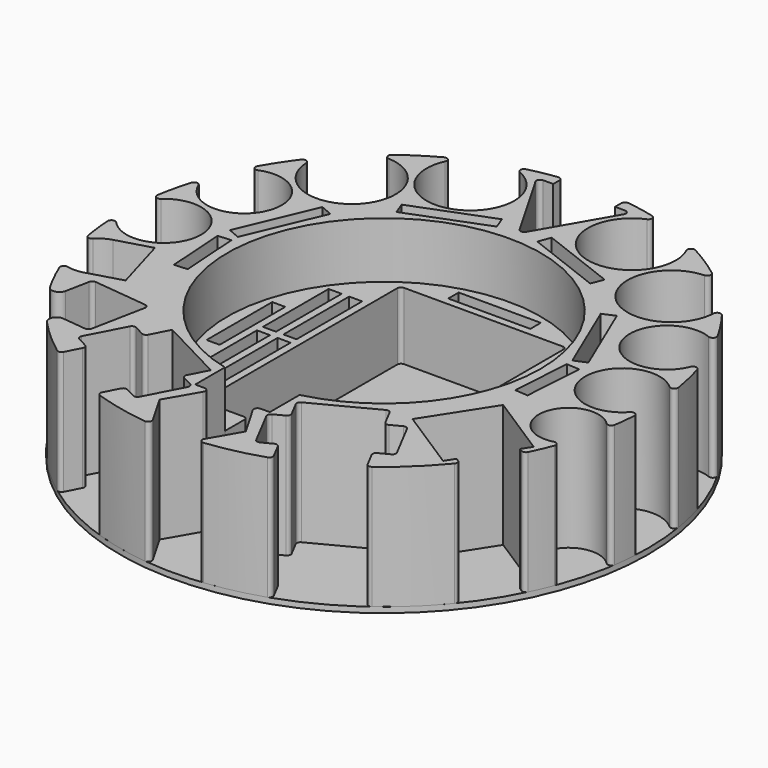
from build123d import *

# Parameters (mm, degrees)
F0_W     = 3.5
F0_H     = 22
F0_W_2   = 22
F0_H_2   = 3.5
F1_DEPTH = 18
F2_R     = 1
F3_DEPTH = 33
F4_R     = 1
F5_DEPTH = 5
F6_R     = 2
F7_R     = 70.7060990639
F8_DEPTH = 1.5


# Not quite as in the source:
# - a feature names something its author has since deleted; it is built from what else it names


with BuildPart() as f1:
    # F0 (on Top) → F1 (new body)
    with BuildSketch(Plane.XY):
        with BuildLine():
            Line((-22.25, -33.25), (-22.25, 33.25))
            Line((-22.25, 33.25), (22.25, 33.25))
            Line((22.25, 33.25), (22.25, -33.25))
            Line((22.25, -33.25), (10, -33.25))
            Line((10, -33.25), (10, -40.7921561087))
            ThreePointArc((10, -40.7921561087), (33.0454232837, -25.9229627936), (42, 0))
            ThreePointArc((42, 0), (-25.9229627936, 33.0454232837), (-10, -40.7921561087))
            Line((-10, -40.7921561087), (-10, -33.25))
            Line((-10, -33.25), (-22.25, -33.25))
        make_face()
        with Locations((-31.5, -12)):
            Rectangle(F0_W, F0_H, mode=Mode.SUBTRACT)
        with Locations((-26, -12)):
            Rectangle(F0_W, F0_H, mode=Mode.SUBTRACT)
        with Locations((26, -12)):
            Rectangle(F0_W, F0_H, mode=Mode.SUBTRACT)
        with Locations((31.5, -12)):
            Rectangle(F0_W, F0_H, mode=Mode.SUBTRACT)
        with Locations((-37, 0)):
            Rectangle(F0_W, F0_H, mode=Mode.SUBTRACT)
        with Locations((-31.5, 12)):
            Rectangle(F0_W, F0_H, mode=Mode.SUBTRACT)
        with Locations((-26, 12)):
            Rectangle(F0_W, F0_H, mode=Mode.SUBTRACT)
        with Locations((26, 12)):
            Rectangle(F0_W, F0_H, mode=Mode.SUBTRACT)
        with Locations((31.5, 12)):
            Rectangle(F0_W, F0_H, mode=Mode.SUBTRACT)
        with Locations((37, 0)):
            Rectangle(F0_W, F0_H, mode=Mode.SUBTRACT)
        with Locations((0, 37)):
            Rectangle(F0_W_2, F0_H_2, mode=Mode.SUBTRACT)
    extrude(amount=F1_DEPTH)

    # F2
    f2_edges = [f1.edges().sort_by_distance(p)[0] for p in [
        (-22.25, 33.25, 9),
        (22.25, 33.25, 9),
        (-22.25, -33.25, 9),
        (-10, -33.25, 9),
        (10, -33.25, 9),
        (22.25, -33.25, 9),
    ]]
    fillet(f2_edges, radius=F2_R)


with BuildPart() as f3:
    # F0 (on Top) → F3 (new body)
    with BuildSketch(Plane.XY):
        with BuildLine():
            Line((-10, -50.75), (-10, -40.7921561087))
            ThreePointArc((-10, -40.7921561087), (-25.9229627936, 33.0454232837), (42, 0))
            ThreePointArc((42, 0), (33.0454232837, -25.9229627936), (10, -40.7921561087))
            Line((10, -40.7921561087), (10, -50.75))
            Line((10, -50.75), (5.7735026919, -50.75))
            Line((5.7735026919, -50.75), (11.5470053838, -60.75))
            Line((11.5470053838, -60.75), (5.9405307391, -70.4606989359))
            ThreePointArc((5.9405307391, -70.4606989359), (14.8578112207, -69.1320869476), (23.5335539083, -66.6796208781))
            Line((23.5335539083, -66.6796208781), (20.5251654312, -60.917711579))
            Line((20.5251654312, -60.917711579), (16.0929275088, -63.2318565614))
            Line((16.0929275088, -63.2318565614), (10.0761505547, -51.7080379632))
            Line((10.0761505547, -51.7080379632), (14.5083884771, -49.3938929808))
            Line((14.5083884771, -49.3938929808), (11.5, -43.6319836817))
            Line((11.5, -43.6319836817), (29.2289516895, -34.3754037523))
            Line((29.2289516895, -34.3754037523), (32.2373401666, -40.1373130514))
            Line((32.2373401666, -40.1373130514), (36.669578089, -37.823168069))
            Line((36.669578089, -37.823168069), (42.6863550431, -49.3469866672))
            Line((42.6863550431, -49.3469866672), (38.2541171207, -51.6611316496))
            Line((38.2541171207, -51.6611316496), (41.2625055978, -57.4230409487))
            ThreePointArc((41.2625055978, -57.4230409487), (48.8073571862, -51.1648500877), (55.4142315383, -43.9233758153))
            Line((55.4142315383, -43.9233758153), (53.7315938597, -42.8422974451))
            Line((53.7315938597, -42.8422974451), (52.1099763044, -45.366253963))
            Line((52.1099763044, -45.366253963), (35.2835995184, -34.5554702609))
            Line((35.2835995184, -34.5554702609), (46.0943832206, -17.7290934748))
            Line((46.0943832206, -17.7290934748), (62.9207600066, -28.539877177))
            Line((62.9207600066, -28.539877177), (61.2991424513, -31.0638336949))
            Line((61.2991424513, -31.0638336949), (62.9817801299, -32.1449120651))
            ThreePointArc((62.9817801299, -32.1449120651), (65.0361749759, -27.7542058885), (66.7849149022, -23.2330613892))
            ThreePointArc((66.7849149022, -23.2330613892), (54.854769381, -14.3894158613), (69.5897634292, -12.5405273363))
            ThreePointArc((69.5897634292, -12.5405273363), (70.3991456201, -6.630256101), (70.7074773009, -0.6727954691))
            ThreePointArc((70.7074773009, -0.6727954691), (51.4368081392, 2.5504447549), (70.2940942413, 7.6642230397))
            ThreePointArc((70.2940942413, 7.6642230397), (68.9245199116, 15.7927374119), (66.6182823129, 23.7066332845))
            ThreePointArc((66.6182823129, 23.7066332845), (47.4157256224, 20.0997254632), (63.3604638504, 31.3919037439))
            ThreePointArc((63.3604638504, 31.3919037439), (59.240304552, 38.6081120567), (54.3020440522, 45.2911471676))
            ThreePointArc((54.3020440522, 45.2911471676), (54.5147403937, 44.0153578981), (54.5859266913, 42.7239205188))
            ThreePointArc((54.5859266913, 42.7239205188), (33.6549667649, 35.390948759), (45.4331650181, 54.1832770921))
            ThreePointArc((45.4331650181, 54.1832770921), (38.1813686703, 59.5162422072), (30.3108121851, 63.8846982045))
            ThreePointArc((30.3108121851, 63.8846982045), (32.5863139632, 60.2120880478), (33.3806107166, 55.9653167598))
            ThreePointArc((33.3806107166, 55.9653167598), (13.7197698433, 47.2773309933), (20.5327644734, 67.6639164037))
            ThreePointArc((20.5327644734, 67.6639164037), (14.4626826133, 69.2158277537), (8.2790561914, 70.224335017))
            Line((8.2790561914, 70.224335017), (8.2790561914, 68))
            Line((8.2790561914, 68), (13.2790561914, 68))
            Line((13.2790561914, 68), (12.7017059222, 67))
            Line((12.7017059222, 67), (0, 45))
            Line((0, 45), (-12.7017059222, 67))
            Line((-12.7017059222, 67), (-13.2790561914, 68))
            Line((-13.2790561914, 68), (-8.2790561914, 68))
            Line((-8.2790561914, 68), (-8.2790561914, 70.224335017))
            ThreePointArc((-8.2790561914, 70.224335017), (-14.4626826133, 69.2158277537), (-20.5327644734, 67.6639164037))
            ThreePointArc((-20.5327644734, 67.6639164037), (-12.9426249501, 63.876157633), (-9.8806107166, 55.9653167598))
            ThreePointArc((-9.8806107166, 55.9653167598), (-25.8773820046, 45.0096135132), (-30.3108121851, 63.8846982045))
            ThreePointArc((-30.3108121851, 63.8846982045), (-38.1813686703, 59.5162422072), (-45.4331650181, 54.1832770921))
            ThreePointArc((-45.4331650181, 54.1832770921), (-35.5029549315, 51.9048804452), (-31.0859266913, 42.7239205188))
            ThreePointArc((-31.0859266913, 42.7239205188), (-44.1273640706, 31.0451068164), (-54.3020440522, 45.2911471676))
            ThreePointArc((-54.3020440522, 45.2911471676), (-59.240304552, 38.6081120567), (-63.3604638504, 31.3919037439))
            ThreePointArc((-63.3604638504, 31.3919037439), (-52.5839754821, 33.1507543239), (-46.6226626365, 24.0025847765))
            ThreePointArc((-46.6226626365, 24.0025847765), (-56.4746706833, 14.0036799174), (-66.6182823129, 23.7066332845))
            ThreePointArc((-66.6182823129, 23.7066332845), (-68.9245199116, 15.7927374119), (-70.2940942413, 7.6642230397))
            ThreePointArc((-70.2940942413, 7.6642230397), (-59.0470984607, 12.7589553806), (-51.424537875, 3.0456767461))
            ThreePointArc((-51.424537875, 3.0456767461), (-59.5310482736, -6.7734218444), (-70.7074773009, -0.6727954691))
            ThreePointArc((-70.7074773009, -0.6727954691), (-70.3102260084, -7.5147933206), (-69.252470002, -14.2861960866))
            ThreePointArc((-69.252470002, -14.2861960866), (-67.2261990225, -11.7961041857), (-64.3841434366, -10.3031032469))
            Line((-64.3841434366, -10.3031032469), (-55.2585487166, -7.6623607362))
            Line((-55.2585487166, -7.6623607362), (-50.8109823828, -23.0317834224))
            Line((-50.8109823828, -23.0317834224), (-59.9365771027, -25.6725259331))
            ThreePointArc((-59.9365771027, -25.6725259331), (-63.1367427992, -25.9280083632), (-66.1796753352, -24.9048303051))
            ThreePointArc((-66.1796753352, -24.9048303051), (-62.8198604821, -32.4602083944), (-58.6010205488, -39.5717120003))
            Line((-58.6010205488, -39.5717120003), (-56.1875473689, -27.3716919584))
            Line((-56.1875473689, -27.3716919584), (-39.6843310996, -29.1616228984))
            Line((-39.6843310996, -29.1616228984), (-42.9058008837, -45.4460366867))
            Line((-42.9058008837, -45.4460366867), (-55.2697442136, -44.1050493092))
            ThreePointArc((-55.2697442136, -44.1050493092), (-48.7233110404, -51.2448920504), (-41.2625055978, -57.4230409487))
            Line((-41.2625055978, -57.4230409487), (-38.2541171207, -51.6611316496))
            Line((-38.2541171207, -51.6611316496), (-42.6863550431, -49.3469866672))
            Line((-42.6863550431, -49.3469866672), (-36.669578089, -37.823168069))
            Line((-36.669578089, -37.823168069), (-32.2373401666, -40.1373130514))
            Line((-32.2373401666, -40.1373130514), (-29.2289516895, -34.3754037523))
            Line((-29.2289516895, -34.3754037523), (-11.5, -43.6319836817))
            Line((-11.5, -43.6319836817), (-14.5083884771, -49.3938929808))
            Line((-14.5083884771, -49.3938929808), (-10.0761505547, -51.7080379632))
            Line((-10.0761505547, -51.7080379632), (-16.0929275088, -63.2318565614))
            Line((-16.0929275088, -63.2318565614), (-20.5251654312, -60.917711579))
            Line((-20.5251654312, -60.917711579), (-23.5335539083, -66.6796208781))
            ThreePointArc((-23.5335539083, -66.6796208781), (-14.8578112207, -69.1320869476), (-5.9405307391, -70.4606989359))
            Line((-5.9405307391, -70.4606989359), (-11.5470053838, -60.75))
            Line((-11.5470053838, -60.75), (-5.7735026919, -50.75))
            Line((-5.7735026919, -50.75), (-10, -50.75))
        make_face()
        Polygon((-47.3671913283, -11.1511966026), (-48.4234069114, 4.813903104), (-44.9310413506, 5.0449502628), (-43.8748257675, -10.9201494438), align=None, mode=Mode.SUBTRACT)
        Polygon((44.9310413506, 5.0449502628), (48.4234069114, 4.813903104), (47.3671913283, -11.1511966026), (43.8748257675, -10.9201494438), align=None, mode=Mode.SUBTRACT)
        Polygon((-39.4398055722, 28.6662124534), (-36.2173776173, 27.3002116938), (-44.8036681065, 7.0449502628), (-48.0260960614, 8.4109510225), align=None, mode=Mode.SUBTRACT)
        Polygon((-27.2042864673, 39.8738861638), (-6.683670322, 47.8051100932), (-5.4218846969, 44.5404666156), (-25.9425008421, 36.6092426862), align=None, mode=Mode.SUBTRACT)
        Polygon((36.2173776173, 27.3002116938), (39.4398055722, 28.6662124534), (48.0260960614, 8.4109510225), (44.8036681065, 7.0449502628), align=None, mode=Mode.SUBTRACT)
        Polygon((6.683670322, 47.8051100932), (27.2042864673, 39.8738861638), (25.9425008421, 36.6092426862), (5.4218846969, 44.5404666156), align=None, mode=Mode.SUBTRACT)
        Polygon((-8.2790561914, 67), (-8.2790561914, 68), (-13.2790561914, 68), (-12.7017059222, 67), align=None)
        Polygon((13.2790561914, 68), (8.2790561914, 68), (8.2790561914, 67), (12.7017059222, 67), align=None)
    extrude(amount=F3_DEPTH)

    # F4
    f4_edges = [f3.edges().sort_by_distance(p)[0] for p in [
        (-8.279056, 70.224335, 16.5),
        (8.279056, 70.224335, 16.5),
        (62.98178, -32.144912, 16.5),
        (55.414232, -43.923376, 16.5),
        (66.618282, 23.706633, 16.5),
        (70.294094, 7.664223, 16.5),
        (63.360464, 31.391904, 16.5),
        (54.302044, 45.291147, 16.5),
        (45.433165, 54.183277, 16.5),
        (30.310812, 63.884698, 16.5),
        (20.532764, 67.663916, 16.5),
        (-20.532764, 67.663916, 16.5),
        (-30.310812, 63.884698, 16.5),
        (-45.433165, 54.183277, 16.5),
        (-54.302044, 45.291147, 16.5),
        (-63.360464, 31.391904, 16.5),
        (-66.618282, 23.706633, 16.5),
        (-70.294094, 7.664223, 16.5),
        (-70.707477, -0.672795, 16.5),
        (-69.25247, -14.286196, 16.5),
        (-66.179675, -24.90483, 16.5),
        (-5.940531, -70.460699, 16.5),
        (5.940531, -70.460699, 16.5),
        (66.784915, -23.233061, 16.5),
        (69.589763, -12.540527, 16.5),
        (70.707477, -0.672795, 16.5),
        (-23.533554, -66.679621, 16.5),
        (-41.262506, -57.423041, 16.5),
        (41.262506, -57.423041, 16.5),
        (23.533554, -66.679621, 16.5),
        (5.773503, -50.75, 16.5),
        (-5.773503, -50.75, 16.5),
        (-14.508388, -49.393893, 16.5),
        (-20.525165, -60.917712, 16.5),
        (-16.092928, -63.231857, 16.5),
        (-10.076151, -51.708038, 16.5),
        (-32.23734, -40.137313, 16.5),
        (-38.254117, -51.661132, 16.5),
        (-36.669578, -37.823168, 16.5),
        (-42.686355, -49.346987, 16.5),
        (42.686355, -49.346987, 16.5),
        (16.092928, -63.231857, 16.5),
        (20.525165, -60.917712, 16.5),
        (38.254117, -51.661132, 16.5),
        (36.669578, -37.823168, 16.5),
        (32.23734, -40.137313, 16.5),
        (29.228952, -34.375404, 16.5),
        (11.5, -43.631984, 16.5),
        (14.508388, -49.393893, 16.5),
        (10.076151, -51.708038, 16.5),
        (-12.701706, 67, 16.5),
        (12.701706, 67, 16.5),
        (0, 45, 16.5),
        (-56.187547, -27.371692, 16.5),
        (-39.684331, -29.161623, 16.5),
        (-42.905801, -45.446037, 16.5),
    ]]
    fillet(f4_edges, radius=F4_R)

    # F0 (on Top) → F5 (join)
    with BuildSketch(Plane.XY):
        Polygon((-44.9310413506, 5.0449502628), (-48.4234069114, 4.813903104), (-47.3671913283, -11.1511966026), (-43.8748257675, -10.9201494438), align=None)
        Polygon((-44.8036681065, 7.0449502628), (-36.2173776173, 27.3002116938), (-39.4398055722, 28.6662124534), (-48.0260960614, 8.4109510225), align=None)
        Polygon((-5.4218846969, 44.5404666156), (-6.683670322, 47.8051100932), (-27.2042864673, 39.8738861638), (-25.9425008421, 36.6092426862), align=None)
        Polygon((25.9425008421, 36.6092426862), (27.2042864673, 39.8738861638), (6.683670322, 47.8051100932), (5.4218846969, 44.5404666156), align=None)
        Polygon((48.0260960614, 8.4109510225), (39.4398055722, 28.6662124534), (36.2173776173, 27.3002116938), (44.8036681065, 7.0449502628), align=None)
        Polygon((47.3671913283, -11.1511966026), (48.4234069114, 4.813903104), (44.9310413506, 5.0449502628), (43.8748257675, -10.9201494438), align=None)
    extrude(amount=F5_DEPTH)

    # F6
    f6_edges = [f3.edges().sort_by_distance(p)[0] for p in [
        (-58.601021, -39.571712, 16.5),
        (-55.269744, -44.105049, 16.5),
    ]]
    fillet(f6_edges, radius=F6_R)


with BuildPart() as f8:
    # F7 (on face) → F8 (new body)
    with BuildSketch(Plane(origin=(0, 0, 0), x_dir=(1, 0, 0), z_dir=(0, 0, -1))):
        Circle(F7_R)
    extrude(amount=F8_DEPTH)


solid = Compound([f1.part, f3.part, f8.part])
